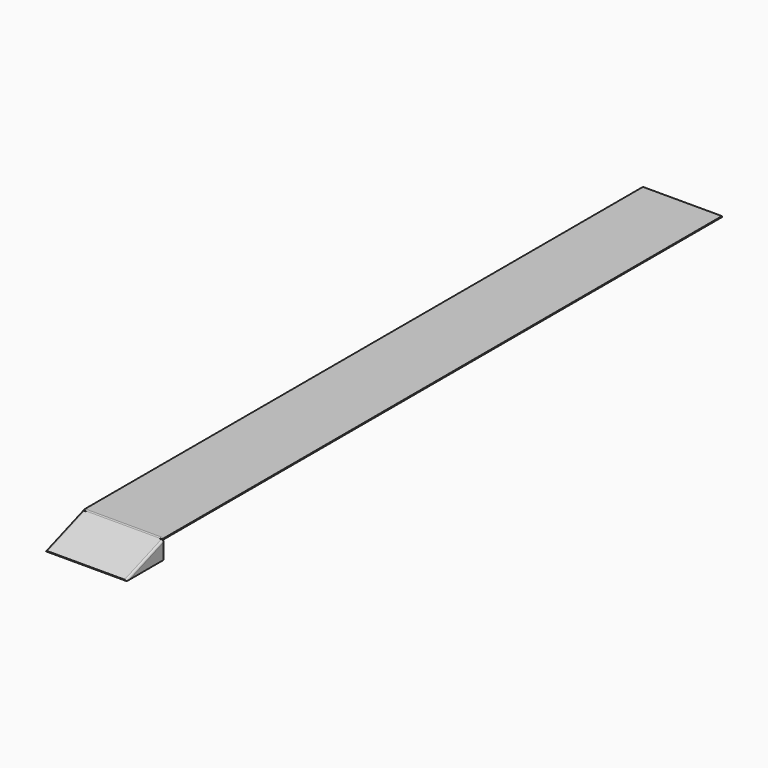
from build123d import *

# Parameters (mm, degrees)
F0_W         = 400
F0_H         = 3530
F1_DEPTH     = 5
F3_DEPTH     = 400
F4_DEPTH     = 250
F6_DEPTH     = 1295.2249255895
F8_DEPTH     = 5
F9_T4_DEPTH  = 298
F9_T9_DEPTH  = 298
F10_T4_DEPTH = 248


# Not quite as in the source:
# - a fillet or chamfer that OpenCascade refuses, or shapes differently, is made with other operations: its cross-section is extruded or revolved along the edge and cut away or added
# - a pattern or mirror of a feature is missing from the dataset's text; its kind, count and spacing are read off the source's solid


with BuildPart() as f1:
    # F0 (on Top) → F1 (new body)
    with BuildSketch(Plane.XY):
        Rectangle(F0_W, F0_H)
    extrude(amount=F1_DEPTH)

    # F2 (on face) → F3 (join, through all)
    with BuildSketch(Plane.YZ.offset(200)):
        with BuildLine():
            Line((-1765, 0), (-1765, 5))
            ThreePointArc((-1765, 5), (-1769.6395282242, 4.4544282326), (-1774.0259368871, 2.8474777857))
            Line((-1774.0259368871, 2.8474777857), (-1772.2994889085, -1.8958990513))
            ThreePointArc((-1772.2994889085, -1.8958990513), (-1768.7708411375, -0.4817095664), (-1765, 0))
        make_face()
    extrude(amount=-F3_DEPTH)

    # F4 (add): a face of the model
    f4_faces = [f1.faces().sort_by_distance(p)[0] for p in [
        (0, -1773.1627128978, 0.4757893672),
    ]]
    extrude(f4_faces, amount=F4_DEPTH)

    # F5 (on face) → F6 (cut, through all)
    with BuildSketch(Plane(origin=(0, -208.4367747126, 572.6753319069), x_dir=(1, 0, 0), z_dir=(0, -0.3420201433, 0.9396926208))):
        with BuildLine():
            Line((200, -1668.0651872152), (200, -1666.0651872152))
            Line((200, -1666.0651872152), (188, -1666.0651872152))
            ThreePointArc((188, -1666.0651872152), (187.6464466094, -1666.2116338246), (187.5, -1666.5651872152))
            Line((187.5, -1666.5651872152), (187.5, -1667.5651872152))
            ThreePointArc((187.5, -1667.5651872152), (187.6464466094, -1667.9187406058), (188, -1668.0651872152))
            Line((188, -1668.0651872152), (200, -1668.0651872152))
        make_face()
        with BuildLine():
            ThreePointArc((-188, -1668.0651872152), (-187.6464466094, -1667.9187406058), (-187.5, -1667.5651872152))
            Line((-187.5, -1667.5651872152), (-187.5, -1666.5651872152))
            ThreePointArc((-187.5, -1666.5651872152), (-187.6464466094, -1666.2116338246), (-188, -1666.0651872152))
            Line((-188, -1666.0651872152), (-200, -1666.0651872152))
            Line((-200, -1666.0651872152), (-200, -1668.0651872152))
            Line((-200, -1668.0651872152), (-188, -1668.0651872152))
        make_face()
    extrude(amount=-F6_DEPTH, mode=Mode.SUBTRACT)

    # F7 (on face) → F8 (join)
    with BuildSketch(Plane.YZ.offset(200)):
        Polygon((-1775.9053221286, 2.163437499), (-2008.9490920835, -82.6575580457), (-2007.222644105, -87.4009348827), (-1774.1788741501, -87.4009348827), (-1774.1788741501, -2.5799393379), align=None)
    f8 = extrude(amount=F8_DEPTH)

    # F8_copies: F8 across plane
    add(f8.mirror(Plane(origin=(0, 0, 0), x_dir=(0, 0, -1), z_dir=(-1, 0, 0))))

    # F9: fillet of radius 10 on 2 edges, made by hand


with BuildPart() as f9_tool2:
    # F9_s3 → F9_t4 (new body)
    with BuildSketch(Plane(origin=(0, -1543.9762318963, -561.9613908248), x_dir=(1, 0, 0), z_dir=(0, -0.9396926208, -0.3420201433))):
        with BuildLine():
            ThreePointArc((205, 599.4283590606), (202.0710678119, 606.4994268725), (195, 609.4283590606))
            Line((195, 609.4283590606), (205, 609.4283590606))
            Line((205, 609.4283590606), (205, 599.4283590606))
        make_face()
    extrude(amount=F9_T4_DEPTH)

    split(bisect_by=Plane(origin=(0, -1565.5891621744, -569.8278541213), x_dir=(1, 0, 0), z_dir=(0, -0.9396926208, -0.3420201433)), keep=Keep.TOP)


with BuildPart() as f1_1:
    add(f1.part)

    # F9_t1: cut F9_tool2
    add(f9_tool2.part, mode=Mode.SUBTRACT)


with BuildPart() as f9_tool7:
    # F9_s8 → F9_t9 (new body)
    with BuildSketch(Plane(origin=(0, -1543.9762318963, -561.9613908248), x_dir=(1, 0, 0), z_dir=(0, -0.9396926208, -0.3420201433))):
        with BuildLine():
            ThreePointArc((-205, 599.4283590606), (-202.0710678119, 606.4994268725), (-195, 609.4283590606))
            Line((-195, 609.4283590606), (-205, 609.4283590606))
            Line((-205, 609.4283590606), (-205, 599.4283590606))
        make_face()
    extrude(amount=F9_T9_DEPTH)

    split(bisect_by=Plane.XZ.offset(1774.1788741501), keep=Keep.TOP)


with BuildPart() as f1_2:
    add(f1_1.part)

    # F9_t6: cut F9_tool7
    add(f9_tool7.part, mode=Mode.SUBTRACT)

    # F10: fillet of radius 5 on 1 edges, made by hand


with BuildPart() as f10_tool2:
    # F10_s3 → F10_t4 (new body)
    with BuildSketch(Plane(origin=(0, -1567.468547416, -570.5118944079), x_dir=(1, 0, 0), z_dir=(0, -0.9396926208, -0.3420201433))):
        with BuildLine():
            ThreePointArc((195, 604.3805628643), (198.5355339059, 602.9160967702), (200, 599.3805628643))
            Line((200, 599.3805628643), (200, 604.3805628643))
            Line((200, 604.3805628643), (195, 604.3805628643))
        make_face()
    extrude(amount=F10_T4_DEPTH)

    split(bisect_by=Plane.XZ.offset(1774.1788741501), keep=Keep.TOP)

    split(bisect_by=Plane.XY.offset(-87.4009348827), keep=Keep.TOP)


with BuildPart() as f1_3:
    add(f1_2.part)

    # F10_t1: union F10_tool2
    add(f10_tool2.part)


solid = f1_3.part
